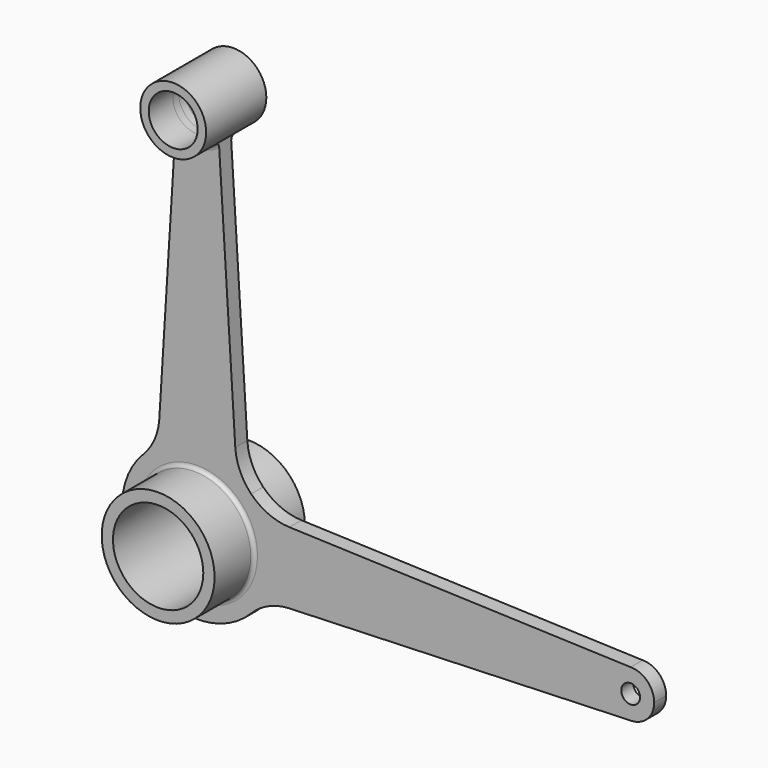
from build123d import *

# Parameters (mm, degrees)
F0_R          = 30
F0_R_2        = 5
F0_R_3        = 13
F1_DEPTH      = 4
F2_R          = 30
F3_T1_DEPTH   = 8
F4_R          = 30
F5_R          = 30
F7_DEPTH      = 20
F6_R          = 30
F6_R_2        = 24
F8_DEPTH      = 30
F9_R          = 2
F10_T4_ANGLE  = 114.9160729666
F10_T10_ANGLE = 114.9160729666


# Not quite as in the source:
# - a fillet or chamfer that OpenCascade refuses, or shapes differently, is made with other operations: its cross-section is extruded or revolved along the edge and cut away or added


with BuildPart() as f1:
    # F0 (on Front) → F1 (new body, symmetric)
    with BuildSketch(Plane.XZ):
        with BuildLine():
            ThreePointArc((34.9249194702, -19.5), (38.7104428986, -10.074800772), (40, 0))
            ThreePointArc((40, 0), (38.7104428986, 10.074800772), (34.9249194702, 19.5))
            ThreePointArc((34.9249194702, 19.5), (28.892590505, 27.6625778609), (21, 34.0440890611))
            ThreePointArc((21, 34.0440890611), (0, 40), (-21, 34.0440890611))
            ThreePointArc((-21, 34.0440890611), (-27.6625778609, -28.892590505), (34.9249194702, -19.5))
        make_face()
        Circle(F0_R, mode=Mode.SUBTRACT)
        with BuildLine():
            ThreePointArc((34.9249194702, 19.5), (38.7104428986, 10.074800772), (40, 0))
            ThreePointArc((40, 0), (38.7104428986, -10.074800772), (34.9249194702, -19.5))
            Line((34.9249194702, -19.5), (230.3062081337, -12.5))
            ThreePointArc((230.3062081337, -12.5), (217.8062081337, 0), (230.3062081337, 12.5))
            Line((230.3062081337, 12.5), (34.9249194702, 19.5))
        make_face()
        with BuildLine():
            ThreePointArc((-21, 34.0440890611), (0, 40), (21, 34.0440890611))
            Line((21, 34.0440890611), (11.5, 186.8090940417))
            ThreePointArc((11.5, 186.8090940417), (0, 182.5), (-11.5, 186.8090940417))
            Line((-11.5, 186.8090940417), (-21, 34.0440890611))
        make_face()
        with BuildLine():
            ThreePointArc((242.8062081337, 0), (239.1450428985, 8.8388347648), (230.3062081337, 12.5))
            ThreePointArc((230.3062081337, 12.5), (217.8062081337, 0), (230.3062081337, -12.5))
            ThreePointArc((230.3062081337, -12.5), (239.1450428985, -8.8388347648), (242.8062081337, 0))
        make_face()
        with Locations((230.3062081337, 0)):
            Circle(F0_R_2, mode=Mode.SUBTRACT)
        with BuildLine():
            ThreePointArc((-11.5, 186.8090940417), (0, 182.5), (11.5, 186.8090940417))
            ThreePointArc((11.5, 186.8090940417), (15.9295323221, 192.7543116269), (17.5, 200))
            ThreePointArc((17.5, 200), (-7.2456883731, 215.9295323221), (-11.5, 186.8090940417))
        make_face()
        with Locations((0, 200)):
            Circle(F0_R_3, mode=Mode.SUBTRACT)
    extrude(amount=F1_DEPTH, both=True)

    # F2
    f2_edges = [f1.edges().sort_by_distance(p)[0] for p in [
        (21, 0, 34.044089),
    ]]
    fillet(f2_edges, radius=F2_R)

    # F3: fillet of radius 30 on 1 edges, made by hand

    # F3_s2 → F3_t1 (join)
    with BuildSketch(Plane.XZ.offset(-4)):
        with BuildLine():
            ThreePointArc((28.5776054959, 27.9878628002), (37.8926630157, 21.5351718891), (48.9366773254, 18.9979954035))
            Line((48.9366773254, 18.9979954035), (34.9249194702, 19.5))
            ThreePointArc((34.9249194702, 19.5), (32.033632685, 23.9550908369), (28.5776054959, 27.9878628002))
        make_face()
    extrude(amount=F3_T1_DEPTH)

    # F4
    f4_edges = [f1.edges().sort_by_distance(p)[0] for p in [
        (-21, 0, 34.044089),
    ]]
    fillet(f4_edges, radius=F4_R)

    # F5
    f5_edges = [f1.edges().sort_by_distance(p)[0] for p in [
        (34.924919, 0, -19.5),
    ]]
    fillet(f5_edges, radius=F5_R)

    # F0 (on Front) → F7 (join, symmetric)
    with BuildSketch(Plane.XZ):
        with BuildLine():
            ThreePointArc((-11.5, 186.8090940417), (0, 182.5), (11.5, 186.8090940417))
            ThreePointArc((11.5, 186.8090940417), (15.9295323221, 192.7543116269), (17.5, 200))
            ThreePointArc((17.5, 200), (-7.2456883731, 215.9295323221), (-11.5, 186.8090940417))
        make_face()
        with Locations((0, 200)):
            Circle(F0_R_3, mode=Mode.SUBTRACT)
    extrude(amount=F7_DEPTH, both=True)

    # F6 (on Front) → F8 (join, symmetric)
    with BuildSketch(Plane.XZ):
        Circle(F6_R)
        Circle(F6_R_2, mode=Mode.SUBTRACT)
    extrude(amount=F8_DEPTH, both=True)

    # F9
    f9_edges = [f1.edges().sort_by_distance(p)[0] for p in [
        (-30, -4, 0),
        (-30, 4, 0),
    ]]
    fillet(f9_edges, radius=F9_R)

    # F10: fillet of radius 2 on 2 edges, made by hand


with BuildPart() as f10_tool2:
    # F10_s3 → F10_t4 (revolve)
    with BuildSketch(Plane(origin=(-90.6925867032, 0, 142.1290246396), x_dir=(0, 1, 0), z_dir=(-0.5379171654, 0, 0.8429977006))):
        with BuildLine():
            ThreePointArc((4, -88.0834330744), (4.5857864376, -89.4976466368), (6, -90.0834330744))
            Line((6, -90.0834330744), (4, -90.0834330744))
            Line((4, -90.0834330744), (4, -88.0834330744))
        make_face()
    revolve(axis=Axis((0, 4, 200), (0, -1, 0)), revolution_arc=F10_T4_ANGLE)

    split(bisect_by=Plane(origin=(-23.028045717, 0, 1.4320454762), x_dir=(0, 1, 0), z_dir=(0.9980719777, 0, -0.0620671193)), keep=Keep.TOP)

    split(bisect_by=Plane(origin=(23.028045717, 0, 1.4320454762), x_dir=(0, 1, 0), z_dir=(-0.9980719777, 0, -0.0620671193)), keep=Keep.TOP)


with BuildPart() as f1_1:
    add(f1.part)

    # F10_t1: union F10_tool2
    add(f10_tool2.part)


with BuildPart() as f10_tool8:
    # F10_s9 → F10_t10 (revolve)
    with BuildSketch(Plane(origin=(90.6925867032, 0, 142.1290246396), x_dir=(0, 1, 0), z_dir=(0.5379171654, 0, 0.8429977006))):
        with BuildLine():
            ThreePointArc((-4, 88.0834330744), (-4.5857864376, 89.4976466368), (-6, 90.0834330744))
            Line((-6, 90.0834330744), (-4, 90.0834330744))
            Line((-4, 90.0834330744), (-4, 88.0834330744))
        make_face()
    revolve(axis=Axis((0, -4, 200), (0, 1, 0)), revolution_arc=F10_T10_ANGLE)

    split(bisect_by=Plane(origin=(-23.028045717, 0, 1.4320454762), x_dir=(0, 1, 0), z_dir=(0.9980719777, 0, -0.0620671193)), keep=Keep.TOP)

    split(bisect_by=Plane(origin=(23.028045717, 0, 1.4320454762), x_dir=(0, 1, 0), z_dir=(-0.9980719777, 0, -0.0620671193)), keep=Keep.TOP)


with BuildPart() as f1_2:
    add(f1_1.part)

    # F10_t7: union F10_tool8
    add(f10_tool8.part)


solid = f1_2.part
